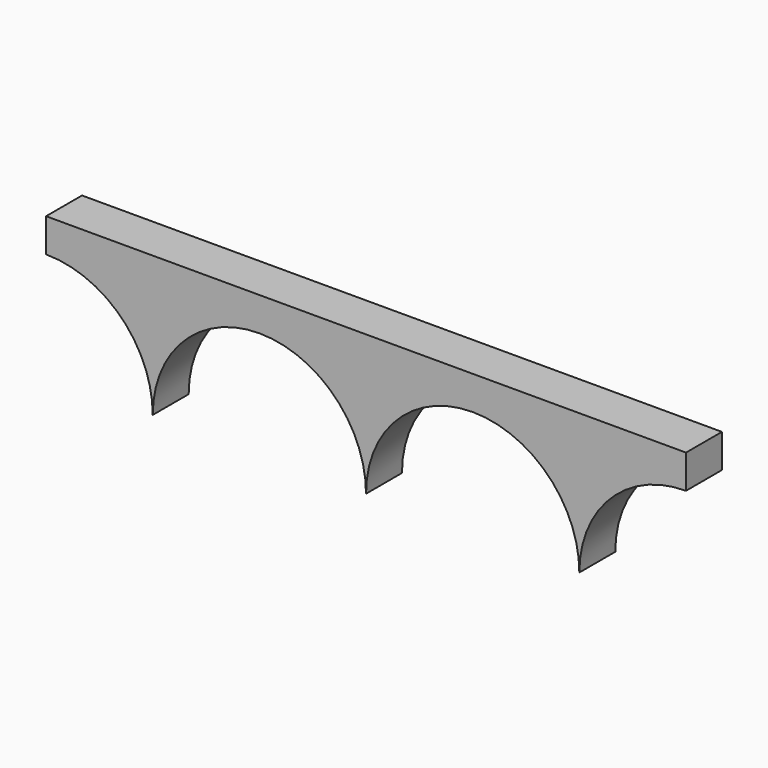
from build123d import *

# Parameters (mm, degrees)
F1_DEPTH = 12.7


# Not quite as in the source:
# - ends of sketch curves that miss each other by under 0.0002 mm in the source are joined


with BuildPart() as f1:
    # F0 (on Front) → F1 (new body)
    with BuildSketch(Plane.XZ):
        with BuildLine():
            Line((90.4875, -9.1365433148), (-90.4875, -9.1365433148))
            Line((-90.4875, -9.1365433148), (-90.4875, -18.6488433148))
            ThreePointArc((-90.4875, -18.6488433148), (-69.1593908483, -27.4832345546), (-60.3249986632, -48.8113433148))
            ThreePointArc((-60.3249986632, -48.8113433148), (-30.1625, -18.6615433148), (-2.6737e-06, -48.8113433154))
            ThreePointArc((-2.6737e-06, -48.8113433154), (30.1625, -18.6488433148), (60.325, -48.8113433148))
            ThreePointArc((60.325, -48.8113433148), (69.1593917125, -27.4832350273), (90.4875, -18.6488433148))
            Line((90.4875, -18.6488433148), (90.4875, -9.1365433148))
        make_face()
    extrude(amount=F1_DEPTH)


solid = f1.part
